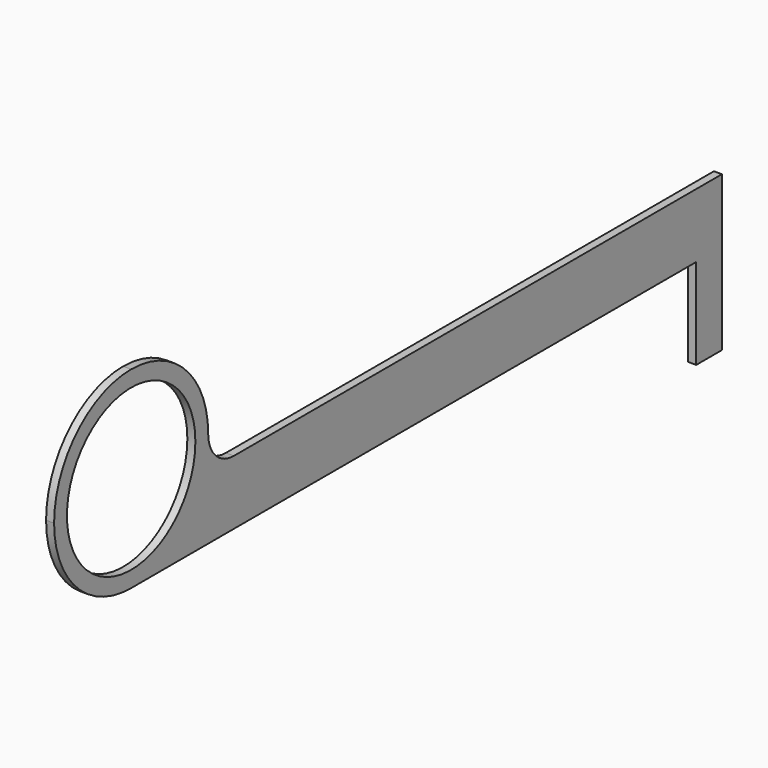
from build123d import *

# Parameters (mm, degrees)
F1_DEPTH = 1.5875
F2_R     = 19.04999
F3_R     = 6.35
F4_R     = 15.875
F5_DEPTH = 25.4


# Not quite as in the source:
# - a fillet or chamfer is up to 0.001 mm smaller than in the source, because OpenCascade refuses the exact size


with BuildPart() as f1:
    # F0 (on Right) → F1 (new body)
    with BuildSketch(Plane.YZ):
        Polygon((-77.51046875, 16.5875132085), (81.23953125, 16.5875132085), (81.23953125, -1.3419014323), (87.58953125, -1.3419014323), (87.58953125, 29.2875132085), (-39.41046875, 29.2875132085), (-39.41046875, 54.6875132085), (-77.51046875, 54.6875132085), align=None)
    extrude(amount=F1_DEPTH)

    # F2 (radius 19.05 in the source; OpenCascade refuses exactly that, so slightly less here)
    f2_edges = [f1.edges().sort_by_distance(p)[0] for p in [
        (0.79375, -77.510469, 54.687513),
        (0.79375, -77.510469, 16.587513),
        (0.79375, -39.410469, 54.687513),
    ]]
    fillet(f2_edges, radius=F2_R)

    # F3
    f3_edges = [f1.edges().sort_by_distance(p)[0] for p in [
        (0.79375, -39.410469, 29.287513),
    ]]
    fillet(f3_edges, radius=F3_R)

    # F4 (on face) → F5 (cut)
    with BuildSketch(Plane.YZ.offset(1.5875)):
        with Locations((-58.46046875, 35.6375132085)):
            Circle(F4_R)
    extrude(amount=-F5_DEPTH, mode=Mode.SUBTRACT)


solid = f1.part
